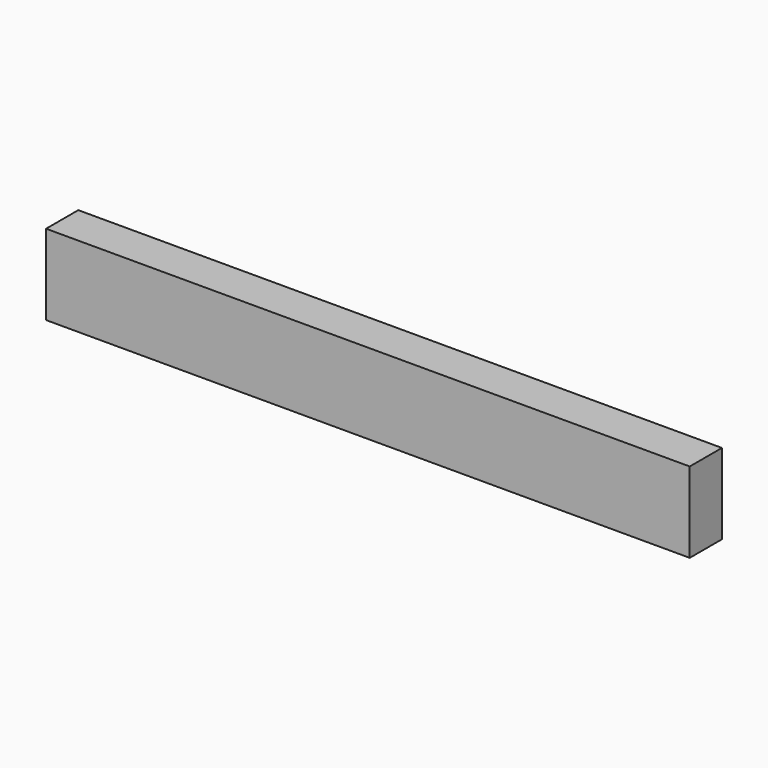
from build123d import *

# Parameters (mm, degrees)
F0_W     = 25.4
F0_H     = 1.5875
F1_DEPTH = 3.175


# Not quite as in the source:
# - a length typed as a fraction of an inch, garbled in the dataset ("3 / 203.2 mm" for 3/8 in), is restored


with BuildPart() as f1:
    # F0 (on Top) → F1 (new body)
    with BuildSketch(Plane.XY):
        Rectangle(F0_W, F0_H)
    extrude(amount=F1_DEPTH)


solid = f1.part
